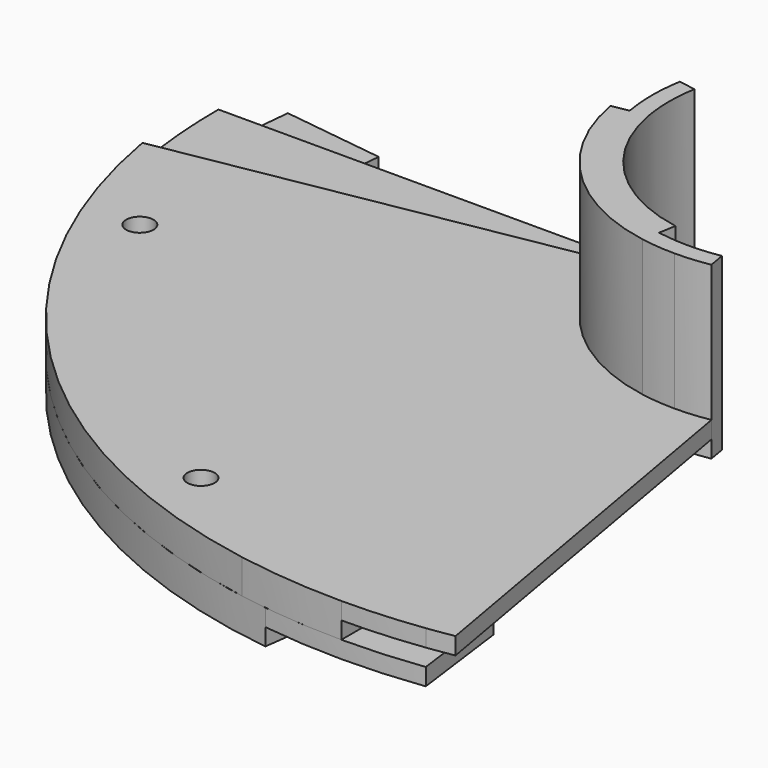
from build123d import *

# Parameters (mm, degrees)
F0_R      = 4.953
F0_R_2    = 3.683
F0_R_3    = 2.54
F1_DEPTH  = 6.35
F2_DEPTH  = 3.175
F3_DEPTH  = 6.35
F4_DEPTH  = 3.175
F5_DEPTH  = 3.556
F6_DEPTH  = 3.556
F7_DEPTH  = 5.334
F8_DEPTH  = 5.334
F9_DEPTH  = 25.4
F10_R     = 2.54
F11_DEPTH = 6.35
F12_DEPTH = 31.75
F13_DEPTH = 6.35
F14_DEPTH = 3.175
F15_DEPTH = 6.35
F16_DEPTH = 3.175


with BuildPart() as f1:
    # F0 (on Top) → F1 (new body)
    with BuildSketch(Plane.XY):
        with BuildLine():
            Line((-94.4351230459, -12.432619809), (-113.322147655, -14.9191437708))
            ThreePointArc((-113.322147655, -14.9191437708), (-80.8223050896, -80.8223050896), (-14.9191437708, -113.322147655))
            Line((-14.9191437708, -113.322147655), (-12.432619809, -94.4351230459))
            ThreePointArc((-12.432619809, -94.4351230459), (-67.351920908, -67.351920908), (-94.4351230459, -12.432619809))
        make_face()
        with Locations((-40.0956566261, -96.7994780189)):
            Circle(F0_R, mode=Mode.SUBTRACT)
        with Locations((-96.7618797455, -40.1863067863)):
            Circle(F0_R, mode=Mode.SUBTRACT)
        with Locations((-96.7618797455, -40.1863067863)):
            Circle(F0_R)
        with Locations((-96.7618797455, -40.1863067863)):
            Circle(F0_R_2, mode=Mode.SUBTRACT)
        with Locations((-96.7618797455, -40.1863067863)):
            Circle(F0_R_2)
        with Locations((-96.7618797455, -40.1863067863)):
            Circle(F0_R_3, mode=Mode.SUBTRACT)
        with Locations((-40.0956566261, -96.7994780189)):
            Circle(F0_R)
        with Locations((-40.0956566261, -96.7994780189)):
            Circle(F0_R_2, mode=Mode.SUBTRACT)
        with Locations((-40.0956566261, -96.7994780189)):
            Circle(F0_R_2)
        with Locations((-40.0956566261, -96.7994780189)):
            Circle(F0_R_3, mode=Mode.SUBTRACT)
    extrude(amount=F1_DEPTH)

    # F0 (on Top) → F2 (join)
    with BuildSketch(Plane.XY):
        with BuildLine():
            Line((-94.4351230459, 12.432619809), (-113.322147655, 14.9191437708))
            ThreePointArc((-113.322147655, 14.9191437708), (-114.3, 0), (-113.322147655, -14.9191437708))
            Line((-113.322147655, -14.9191437708), (-94.4351230459, -12.432619809))
            ThreePointArc((-94.4351230459, -12.432619809), (-95.25, 0), (-94.4351230459, 12.432619809))
        make_face()
        with Locations((-104.775, 0)):
            Circle(F0_R_3, mode=Mode.SUBTRACT)
    extrude(amount=F2_DEPTH)

    # F0 (on Top) → F3 (join)
    with BuildSketch(Plane.XY):
        with BuildLine():
            ThreePointArc((-14.9191437708, -113.322147655), (0, -114.3), (14.9191437708, -113.322147655))
            Line((14.9191437708, -113.322147655), (12.432619809, -94.4351230459))
            ThreePointArc((12.432619809, -94.4351230459), (0, -95.25), (-12.432619809, -94.4351230459))
            Line((-12.432619809, -94.4351230459), (-14.9191437708, -113.322147655))
        make_face()
        with Locations((0, -104.775)):
            Circle(F0_R_3, mode=Mode.SUBTRACT)
    extrude(amount=F3_DEPTH)

    # F0 (on Top) → F4 (cut)
    with BuildSketch(Plane.XY):
        with BuildLine():
            ThreePointArc((-14.9191437708, -113.322147655), (0, -114.3), (14.9191437708, -113.322147655))
            Line((14.9191437708, -113.322147655), (12.432619809, -94.4351230459))
            ThreePointArc((12.432619809, -94.4351230459), (0, -95.25), (-12.432619809, -94.4351230459))
            Line((-12.432619809, -94.4351230459), (-14.9191437708, -113.322147655))
        make_face()
        with Locations((0, -104.775)):
            Circle(F0_R_3, mode=Mode.SUBTRACT)
    extrude(amount=F4_DEPTH, mode=Mode.SUBTRACT)

    # F0 (on Top) → F5 (cut)
    with BuildSketch(Plane.XY):
        with Locations((-40.0956566261, -96.7994780189)):
            Circle(F0_R)
        with Locations((-40.0956566261, -96.7994780189)):
            Circle(F0_R_2, mode=Mode.SUBTRACT)
        with Locations((-40.0956566261, -96.7994780189)):
            Circle(F0_R_2)
        with Locations((-40.0956566261, -96.7994780189)):
            Circle(F0_R_3, mode=Mode.SUBTRACT)
    extrude(amount=F5_DEPTH, mode=Mode.SUBTRACT)

    # F0 (on Top) → F6 (cut)
    with BuildSketch(Plane.XY):
        with Locations((-96.7618797455, -40.1863067863)):
            Circle(F0_R)
        with Locations((-96.7618797455, -40.1863067863)):
            Circle(F0_R_2, mode=Mode.SUBTRACT)
        with Locations((-96.7618797455, -40.1863067863)):
            Circle(F0_R_2)
        with Locations((-96.7618797455, -40.1863067863)):
            Circle(F0_R_3, mode=Mode.SUBTRACT)
    extrude(amount=F6_DEPTH, mode=Mode.SUBTRACT)

    # F0 (on Top) → F7 (cut)
    with BuildSketch(Plane.XY):
        with Locations((-96.7618797455, -40.1863067863)):
            Circle(F0_R_2)
        with Locations((-96.7618797455, -40.1863067863)):
            Circle(F0_R_3, mode=Mode.SUBTRACT)
    extrude(amount=F7_DEPTH, mode=Mode.SUBTRACT)

    # F0 (on Top) → F8 (cut)
    with BuildSketch(Plane.XY):
        with Locations((-40.0956566261, -96.7994780189)):
            Circle(F0_R_2)
        with Locations((-40.0956566261, -96.7994780189)):
            Circle(F0_R_3, mode=Mode.SUBTRACT)
    extrude(amount=F8_DEPTH, mode=Mode.SUBTRACT)

    # F0 (on Top) → F9 (cut)
    with BuildSketch(Plane.XY):
        with Locations((-96.7618797455, -40.1863067863)):
            Circle(F0_R_3)
    extrude(amount=F9_DEPTH, mode=Mode.SUBTRACT)


with BuildPart() as f11:
    # F10 (on face) → F11 (new body)
    with BuildSketch(Plane.XY.offset(6.35)):
        with BuildLine():
            Line((-36.83, 0), (-114.3, 0))
            ThreePointArc((-114.3, 0), (-114.0552749262, -7.475577671), (-113.322147655, -14.9191437708))
            Line((-113.322147655, -14.9191437708), (-94.4351230459, -12.432619809))
            ThreePointArc((-94.4351230459, -12.432619809), (-94.1414338721, -14.4897525346), (-93.8029384744, -16.5399889228))
            Line((-93.8029384744, -16.5399889228), (-36.2704695434, -6.3954623835))
            ThreePointArc((-36.2704695434, -6.3954623835), (-36.6898507307, -3.2099460054), (-36.83, 0))
        make_face()
        with BuildLine():
            Line((-93.8029384744, -16.5399889228), (-112.5635261693, -19.8479867073))
            ThreePointArc((-112.5635261693, -19.8479867073), (-80.8223050896, -80.8223050896), (-19.8479867073, -112.5635261693))
            Line((-19.8479867073, -112.5635261693), (-16.5399889228, -93.8029384744))
            ThreePointArc((-16.5399889228, -93.8029384744), (-67.351920908, -67.351920908), (-93.8029384744, -16.5399889228))
        make_face()
        with Locations((-40.0956566261, -96.7994780189)):
            Circle(F10_R, mode=Mode.SUBTRACT)
        with Locations((-96.7618797455, -40.1863067863)):
            Circle(F10_R, mode=Mode.SUBTRACT)
        with BuildLine():
            ThreePointArc((-6.3954623835, -36.2704695434), (-26.0427427511, -26.0427427511), (-36.2704695434, -6.3954623835))
            Line((-36.2704695434, -6.3954623835), (-93.8029384744, -16.5399889228))
            ThreePointArc((-93.8029384744, -16.5399889228), (-67.351920908, -67.351920908), (-16.5399889228, -93.8029384744))
            Line((-16.5399889228, -93.8029384744), (-6.3954623835, -36.2704695434))
        make_face()
        with BuildLine():
            Line((-33.1437049276, -5.8441294194), (-36.2704695434, -6.3954623835))
            ThreePointArc((-36.2704695434, -6.3954623835), (-26.0427427511, -26.0427427511), (-6.3954623835, -36.2704695434))
            Line((-6.3954623835, -36.2704695434), (-5.8441294194, -33.1437049276))
            ThreePointArc((-5.8441294194, -33.1437049276), (-23.7976787208, -23.7976787208), (-33.1437049276, -5.8441294194))
        make_face()
        with BuildLine():
            Line((-30.0169403118, -5.2927964553), (-33.1437049276, -5.8441294194))
            ThreePointArc((-33.1437049276, -5.8441294194), (-23.7976787208, -23.7976787208), (-5.8441294194, -33.1437049276))
            Line((-5.8441294194, -33.1437049276), (-5.2927964553, -30.0169403118))
            ThreePointArc((-5.2927964553, -30.0169403118), (-21.5526146906, -21.5526146906), (-30.0169403118, -5.2927964553))
        make_face()
        with BuildLine():
            Line((0, -95.25), (0, -36.83))
            ThreePointArc((0, -36.83), (-3.2099460054, -36.6898507307), (-6.3954623835, -36.2704695434))
            Line((-6.3954623835, -36.2704695434), (-16.5399889228, -93.8029384744))
            ThreePointArc((-16.5399889228, -93.8029384744), (-8.3015844967, -94.8875449932), (0, -95.25))
        make_face()
        with BuildLine():
            ThreePointArc((-6.3954623835, -36.2704695434), (-3.2099460054, -36.6898507307), (0, -36.83))
            Line((0, -36.83), (0, -33.655))
            ThreePointArc((0, -33.655), (-2.9332265222, -33.5269325643), (-5.8441294194, -33.1437049276))
            Line((-5.8441294194, -33.1437049276), (-6.3954623835, -36.2704695434))
        make_face()
        with BuildLine():
            Line((-30.48, 0), (-33.655, 0))
            ThreePointArc((-33.655, 0), (-33.5269325643, -2.9332265222), (-33.1437049276, -5.8441294194))
            Line((-33.1437049276, -5.8441294194), (-30.0169403118, -5.2927964553))
            ThreePointArc((-30.0169403118, -5.2927964553), (-30.3640143978, -2.6565070389), (-30.48, 0))
        make_face()
        with BuildLine():
            Line((-94.4351230459, -12.432619809), (-113.322147655, -14.9191437708))
            ThreePointArc((-113.322147655, -14.9191437708), (-112.9697206465, -17.3877030415), (-112.5635261693, -19.8479867073))
            Line((-112.5635261693, -19.8479867073), (-93.8029384744, -16.5399889228))
            ThreePointArc((-93.8029384744, -16.5399889228), (-94.1414338721, -14.4897525346), (-94.4351230459, -12.432619809))
        make_face()
        with BuildLine():
            ThreePointArc((-19.8479867073, -112.5635261693), (-9.9619013961, -113.8650539919), (0, -114.3))
            Line((0, -114.3), (0, -107.315))
            ThreePointArc((0, -107.315), (-2.54, -104.775), (0, -102.235))
            Line((0, -102.235), (0, -95.25))
            ThreePointArc((0, -95.25), (-8.3015844967, -94.8875449932), (-16.5399889228, -93.8029384744))
            Line((-16.5399889228, -93.8029384744), (-19.8479867073, -112.5635261693))
        make_face()
        with BuildLine():
            ThreePointArc((0, -102.235), (-2.54, -104.775), (0, -107.315))
            Line((0, -107.315), (0, -102.235))
        make_face()
    extrude(amount=F11_DEPTH)

    # F10 (on face) → F12 (join)
    with BuildSketch(Plane.XY.offset(6.35)):
        with BuildLine():
            Line((-30.48, 0), (-33.655, 0))
            ThreePointArc((-33.655, 0), (-33.5269325643, -2.9332265222), (-33.1437049276, -5.8441294194))
            Line((-33.1437049276, -5.8441294194), (-30.0169403118, -5.2927964553))
            ThreePointArc((-30.0169403118, -5.2927964553), (-30.3640143978, -2.6565070389), (-30.48, 0))
        make_face()
        with BuildLine():
            Line((-33.1437049276, -5.8441294194), (-36.2704695434, -6.3954623835))
            ThreePointArc((-36.2704695434, -6.3954623835), (-26.0427427511, -26.0427427511), (-6.3954623835, -36.2704695434))
            Line((-6.3954623835, -36.2704695434), (-5.8441294194, -33.1437049276))
            ThreePointArc((-5.8441294194, -33.1437049276), (-23.7976787208, -23.7976787208), (-33.1437049276, -5.8441294194))
        make_face()
        with BuildLine():
            Line((-30.0169403118, -5.2927964553), (-33.1437049276, -5.8441294194))
            ThreePointArc((-33.1437049276, -5.8441294194), (-23.7976787208, -23.7976787208), (-5.8441294194, -33.1437049276))
            Line((-5.8441294194, -33.1437049276), (-5.2927964553, -30.0169403118))
            ThreePointArc((-5.2927964553, -30.0169403118), (-21.5526146906, -21.5526146906), (-30.0169403118, -5.2927964553))
        make_face()
        with BuildLine():
            ThreePointArc((-6.3954623835, -36.2704695434), (-3.2099460054, -36.6898507307), (0, -36.83))
            Line((0, -36.83), (0, -33.655))
            ThreePointArc((0, -33.655), (-2.9332265222, -33.5269325643), (-5.8441294194, -33.1437049276))
            Line((-5.8441294194, -33.1437049276), (-6.3954623835, -36.2704695434))
        make_face()
        with BuildLine():
            Line((-30.0169403118, 5.2927964553), (-33.1437049276, 5.8441294194))
            ThreePointArc((-33.1437049276, 5.8441294194), (-33.5269325643, 2.9332265222), (-33.655, 0))
            Line((-33.655, 0), (-30.48, 0))
            ThreePointArc((-30.48, 0), (-30.3640143978, 2.6565070389), (-30.0169403118, 5.2927964553))
        make_face()
        with BuildLine():
            ThreePointArc((0, -36.83), (3.2099460054, -36.6898507307), (6.3954623835, -36.2704695434))
            Line((6.3954623835, -36.2704695434), (5.8441294194, -33.1437049276))
            ThreePointArc((5.8441294194, -33.1437049276), (2.9332265222, -33.5269325643), (0, -33.655))
            Line((0, -33.655), (0, -36.83))
        make_face()
    extrude(amount=F12_DEPTH)

    # F10 (on face) → F13 (join)
    with BuildSketch(Plane.XY.offset(6.35)):
        with BuildLine():
            Line((0, -102.235), (0, -107.315))
            ThreePointArc((0, -107.315), (1.7960512242, -106.5710512242), (2.54, -104.775))
            ThreePointArc((2.54, -104.775), (1.7960512242, -102.9789487758), (0, -102.235))
        make_face()
        with BuildLine():
            ThreePointArc((0, -114.3), (7.475577671, -114.0552749262), (14.9191437708, -113.322147655))
            Line((14.9191437708, -113.322147655), (12.432619809, -94.4351230459))
            ThreePointArc((12.432619809, -94.4351230459), (6.2296480592, -95.0460624385), (0, -95.25))
            Line((0, -95.25), (0, -102.235))
            ThreePointArc((0, -102.235), (1.7960512242, -102.9789487758), (2.54, -104.775))
            ThreePointArc((2.54, -104.775), (1.7960512242, -106.5710512242), (0, -107.315))
            Line((0, -107.315), (0, -114.3))
        make_face()
        with BuildLine():
            ThreePointArc((14.9191437708, -113.322147655), (17.3877030415, -112.9697206465), (19.8479867073, -112.5635261693))
            Line((19.8479867073, -112.5635261693), (6.3954623835, -36.2704695434))
            ThreePointArc((6.3954623835, -36.2704695434), (3.2099460054, -36.6898507307), (0, -36.83))
            Line((0, -36.83), (0, -95.25))
            ThreePointArc((0, -95.25), (6.2296480592, -95.0460624385), (12.432619809, -94.4351230459))
            Line((12.432619809, -94.4351230459), (14.9191437708, -113.322147655))
        make_face()
    extrude(amount=F13_DEPTH)

    # F10 (on face) → F14 (cut)
    with BuildSketch(Plane.XY.offset(6.35)):
        with BuildLine():
            Line((0, -102.235), (0, -107.315))
            ThreePointArc((0, -107.315), (1.7960512242, -106.5710512242), (2.54, -104.775))
            ThreePointArc((2.54, -104.775), (1.7960512242, -102.9789487758), (0, -102.235))
        make_face()
        with BuildLine():
            ThreePointArc((0, -114.3), (7.475577671, -114.0552749262), (14.9191437708, -113.322147655))
            Line((14.9191437708, -113.322147655), (12.432619809, -94.4351230459))
            ThreePointArc((12.432619809, -94.4351230459), (6.2296480592, -95.0460624385), (0, -95.25))
            Line((0, -95.25), (0, -102.235))
            ThreePointArc((0, -102.235), (1.7960512242, -102.9789487758), (2.54, -104.775))
            ThreePointArc((2.54, -104.775), (1.7960512242, -106.5710512242), (0, -107.315))
            Line((0, -107.315), (0, -114.3))
        make_face()
        with BuildLine():
            ThreePointArc((14.9191437708, -113.322147655), (17.3877030415, -112.9697206465), (19.8479867073, -112.5635261693))
            Line((19.8479867073, -112.5635261693), (6.3954623835, -36.2704695434))
            ThreePointArc((6.3954623835, -36.2704695434), (3.2099460054, -36.6898507307), (0, -36.83))
            Line((0, -36.83), (0, -95.25))
            ThreePointArc((0, -95.25), (6.2296480592, -95.0460624385), (12.432619809, -94.4351230459))
            Line((12.432619809, -94.4351230459), (14.9191437708, -113.322147655))
        make_face()
    extrude(amount=F14_DEPTH, mode=Mode.SUBTRACT)

    # F10 (on face) → F15 (cut)
    with BuildSketch(Plane.XY.offset(6.35)):
        with BuildLine():
            Line((-36.83, 0), (-114.3, 0))
            ThreePointArc((-114.3, 0), (-114.0552749262, -7.475577671), (-113.322147655, -14.9191437708))
            Line((-113.322147655, -14.9191437708), (-94.4351230459, -12.432619809))
            ThreePointArc((-94.4351230459, -12.432619809), (-94.1414338721, -14.4897525346), (-93.8029384744, -16.5399889228))
            Line((-93.8029384744, -16.5399889228), (-36.2704695434, -6.3954623835))
            ThreePointArc((-36.2704695434, -6.3954623835), (-36.6898507307, -3.2099460054), (-36.83, 0))
        make_face()
        with BuildLine():
            Line((-94.4351230459, -12.432619809), (-113.322147655, -14.9191437708))
            ThreePointArc((-113.322147655, -14.9191437708), (-112.9697206465, -17.3877030415), (-112.5635261693, -19.8479867073))
            Line((-112.5635261693, -19.8479867073), (-93.8029384744, -16.5399889228))
            ThreePointArc((-93.8029384744, -16.5399889228), (-94.1414338721, -14.4897525346), (-94.4351230459, -12.432619809))
        make_face()
    extrude(amount=F15_DEPTH, mode=Mode.SUBTRACT)

    # F10 (on face) → F16 (join)
    with BuildSketch(Plane.XY.offset(6.35)):
        with BuildLine():
            Line((-36.83, 0), (-114.3, 0))
            ThreePointArc((-114.3, 0), (-114.0552749262, -7.475577671), (-113.322147655, -14.9191437708))
            Line((-113.322147655, -14.9191437708), (-94.4351230459, -12.432619809))
            ThreePointArc((-94.4351230459, -12.432619809), (-94.1414338721, -14.4897525346), (-93.8029384744, -16.5399889228))
            Line((-93.8029384744, -16.5399889228), (-36.2704695434, -6.3954623835))
            ThreePointArc((-36.2704695434, -6.3954623835), (-36.6898507307, -3.2099460054), (-36.83, 0))
        make_face()
        with BuildLine():
            Line((-94.4351230459, -12.432619809), (-113.322147655, -14.9191437708))
            ThreePointArc((-113.322147655, -14.9191437708), (-112.9697206465, -17.3877030415), (-112.5635261693, -19.8479867073))
            Line((-112.5635261693, -19.8479867073), (-93.8029384744, -16.5399889228))
            ThreePointArc((-93.8029384744, -16.5399889228), (-94.1414338721, -14.4897525346), (-94.4351230459, -12.432619809))
        make_face()
    extrude(amount=F16_DEPTH)


solid = Compound([f1.part, f11.part])
